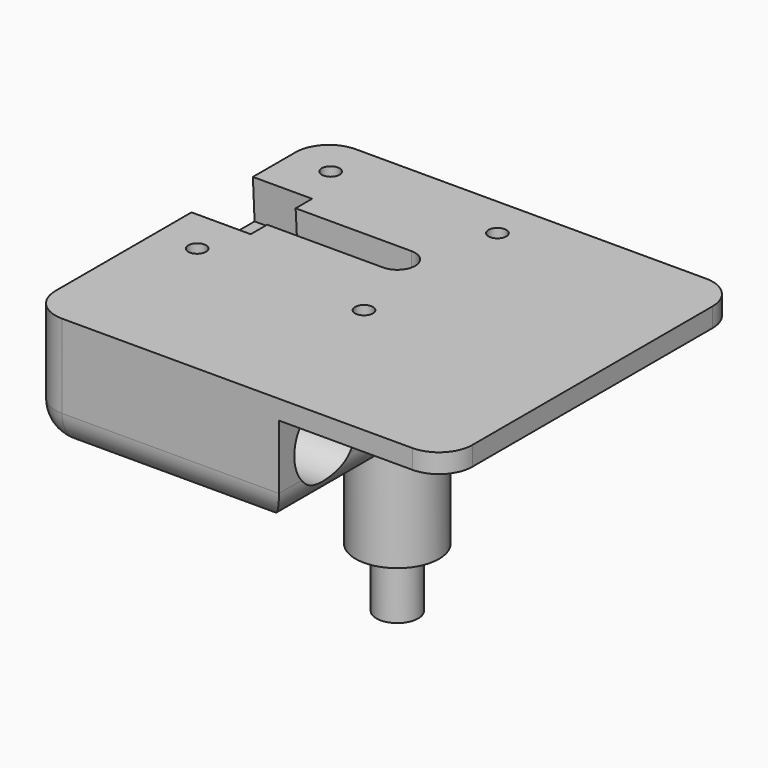
from build123d import *
from build123d import SkipClean  # not in build123d's __all__

# Parameters (mm, degrees)
F0_W          = 38.1
F0_H          = 12.7
F1_DEPTH      = 19.05
F2_W          = 9.017
F2_H          = 3.1369
F2_H_2        = 5.4102
F3_DEPTH      = 6.096
F3_TAPER      = -3
F4_DEPTH      = 4.318
F5_DEPTH      = 12.7010001
F7_R          = 6.35
F7_R_2        = 2.7051
F8_DEPTH      = 25.4
F9_R          = 3.175
F9_R_2        = 2.7051
F10_DEPTH     = 9.017
F11_DEPTH     = 17.78
F12_DEPTH     = 5.08
F14_D         = 11.938
F14_DEPTH     = 25.4
F14_TIP       = 3.586537035
F15_W         = 55.88
F15_H         = 2.921
F16_DEPTH     = 25.4
F17_T1_DEPTH  = 25.4
F17_T3_DEPTH  = 28.321
F17_T5_DEPTH  = 45.72
F17_T7_DEPTH  = 45.72
F17_T9_DEPTH  = 81.28
F17_S13_W     = 5.08
F17_S13_H     = 5.08
F17_T14_DEPTH = 5.08
F17_S19_W     = 5.08
F17_S19_H     = 5.08
F17_T20_DEPTH = 5.08
F18_D         = 2.7051
F18_DEPTH     = 10.16
F18_TIP       = 0.8126940303


# Not quite as in the source:
# - a fillet or chamfer that OpenCascade refuses, or shapes differently, is made with other operations: its cross-section is extruded or revolved along the edge and cut away or added
# - after a boolean that leaves OpenCascade's solid faulty, fix() repairs it


with BuildPart() as f1:
    # F0 (on Front) → F1 (new body, symmetric)
    with BuildSketch(Plane.XZ):
        Rectangle(F0_W, F0_H)
    extrude(amount=F1_DEPTH, both=True)

    # F2 (on face) → F3 (cut)
    with BuildSketch(Plane.XY.offset(6.35)):
        with Locations((-14.5415, 4.27355)):
            Rectangle(F2_W, F2_H)
        with Locations((-14.5415, 0)):
            Rectangle(F2_W, F2_H_2)
        with Locations((-14.5415, -4.27355)):
            Rectangle(F2_W, F2_H)
    extrude(amount=-F3_DEPTH, taper=F3_TAPER, mode=Mode.SUBTRACT)

    # F2 (on face) → F4 (cut)
    with BuildSketch(Plane.XY.offset(6.35)):
        with Locations((-14.5415, 4.27355)):
            Rectangle(F2_W, F2_H)
        with Locations((-14.5415, -4.27355)):
            Rectangle(F2_W, F2_H)
        with BuildLine():
            Line((7.62, 2.7051), (1.8750079208, 2.7051))
            ThreePointArc((1.8750079208, 2.7051), (1.27, 0), (1.8750079208, -2.7051))
            Line((1.8750079208, -2.7051), (7.62, -2.7051))
            ThreePointArc((7.62, -2.7051), (4.9149, 0), (7.62, 2.7051))
        make_face()
        with BuildLine():
            ThreePointArc((1.8750079208, -2.7051), (1.27, 0), (1.8750079208, 2.7051))
            Line((1.8750079208, 2.7051), (-10.033, 2.7051))
            Line((-10.033, 2.7051), (-10.033, -2.7051))
            Line((-10.033, -2.7051), (1.8750079208, -2.7051))
        make_face()
        with Locations((-14.5415, 0)):
            Rectangle(F2_W, F2_H_2)
    extrude(amount=-F4_DEPTH, mode=Mode.SUBTRACT)

    # F2 (on face) → F5 (cut, through all)
    with BuildSketch(Plane.XY.offset(6.35)):
        with BuildLine():
            ThreePointArc((10.3251, 0), (9.5327945538, 1.9127945538), (7.62, 2.7051))
            ThreePointArc((7.62, 2.7051), (4.9149, 0), (7.62, -2.7051))
            ThreePointArc((7.62, -2.7051), (9.5327945538, -1.9127945538), (10.3251, 0))
        make_face()
    extrude(amount=-F5_DEPTH, mode=Mode.SUBTRACT)

    # F7 (on face) → F8 (join)
    with BuildSketch(Plane(origin=(0, 0, -6.35), x_dir=(1, 0, 0), z_dir=(0, 0, -1))):
        with Locations((7.62, 0)):
            Circle(F7_R)
        with Locations((7.62, 0)):
            Circle(F7_R_2, mode=Mode.SUBTRACT)
    with SkipClean():  # cleaning this boolean's faces spoils the solid; the shape is the same uncleaned
        extrude(amount=F8_DEPTH)

    # F9 (on face) → F10 (join)
    with BuildSketch(Plane(origin=(0, 0, -31.75), x_dir=(1, 0, 0), z_dir=(0, 0, -1))):
        with Locations((7.62, 0)):
            Circle(F9_R)
        with Locations((7.62, 0)):
            Circle(F9_R_2, mode=Mode.SUBTRACT)
    extrude(amount=F10_DEPTH)

    add(f1.part.fix(), mode=Mode.REPLACE)

    # F11 (add): a face of the model
    f11_faces = [f1.faces().sort_by_distance(p)[0] for p in [
        (0, -19.05, 0),
    ]]
    extrude(f11_faces, amount=F11_DEPTH)

    # F12 (add): faces of the model
    f12_faces = [f1.faces().sort_by_distance(p)[0] for p in [
        (-0.7285482759, 0, -6.35),
        (0, -27.94, -6.35),
    ]]
    extrude(f12_faces, amount=F12_DEPTH)

    # F14
    with Locations(Plane.YZ.offset(19.05)):
        with Locations((-27.94, -2.54)):
            Hole(F14_D / 2, depth=F14_DEPTH)
            with Locations((0, 0, -(F14_DEPTH + F14_TIP / 2))):  # 118° drill point
                Cone(0, F14_D / 2, F14_TIP, mode=Mode.SUBTRACT)

    # F15 (on face) → F16 (join)
    with BuildSketch(Plane.YZ.offset(19.05)):
        with Locations((-8.89, 4.8895)):
            Rectangle(F15_W, F15_H)
    extrude(amount=F16_DEPTH)

    # F17: fillet of radius 5.08 on 8 edges, made by hand

    # F17_s2 → F17_t1 (cut)
    with BuildSketch(Plane.XY.offset(-6.35)):
        with BuildLine():
            ThreePointArc((-13.97, -36.83), (-17.5621024484, -35.3421024484), (-19.05, -31.75))
            Line((-19.05, -31.75), (-19.05, -36.83))
            Line((-19.05, -36.83), (-13.97, -36.83))
        make_face()
        with BuildLine():
            ThreePointArc((-13.97, 19.05), (-17.5621024484, 17.5621024484), (-19.05, 13.97))
            Line((-19.05, 13.97), (-19.05, 19.05))
            Line((-19.05, 19.05), (-13.97, 19.05))
        make_face()
    extrude(amount=F17_T1_DEPTH, mode=Mode.SUBTRACT)

    # F17_s4 → F17_t3 (cut)
    with BuildSketch(Plane.XY.offset(-9.271)):
        with BuildLine():
            ThreePointArc((39.37, 19.05), (42.9621024484, 17.5621024484), (44.45, 13.97))
            Line((44.45, 13.97), (44.45, 19.05))
            Line((44.45, 19.05), (39.37, 19.05))
        make_face()
        with BuildLine():
            ThreePointArc((44.45, -31.75), (42.9621024484, -35.3421024484), (39.37, -36.83))
            Line((39.37, -36.83), (44.45, -36.83))
            Line((44.45, -36.83), (44.45, -31.75))
        make_face()
    extrude(amount=F17_T3_DEPTH, mode=Mode.SUBTRACT)

    # F17_s6 → F17_t5 (cut)
    with BuildSketch(Plane.XZ.offset(-13.97)):
        with BuildLine():
            ThreePointArc((-13.97, -11.43), (-17.5621024484, -9.9421024484), (-19.05, -6.35))
            Line((-19.05, -6.35), (-19.05, -11.43))
            Line((-19.05, -11.43), (-13.97, -11.43))
        make_face()
    extrude(amount=F17_T5_DEPTH, mode=Mode.SUBTRACT)

    # F17_s8 → F17_t7 (cut)
    with BuildSketch(Plane.YZ.offset(-13.97)):
        with BuildLine():
            ThreePointArc((-31.75, -11.43), (-35.3421024484, -9.9421024484), (-36.83, -6.35))
            Line((-36.83, -6.35), (-36.83, -11.43))
            Line((-36.83, -11.43), (-31.75, -11.43))
        make_face()
        with BuildLine():
            ThreePointArc((13.97, -11.43), (17.5621024484, -9.9421024484), (19.05, -6.35))
            Line((19.05, -6.35), (19.05, -11.43))
            Line((19.05, -11.43), (13.97, -11.43))
        make_face()
    extrude(amount=F17_T7_DEPTH, mode=Mode.SUBTRACT)

    # F17_s10 → F17_t9 (cut)
    with BuildSketch(Plane.XZ.offset(-31.75)):
        with BuildLine():
            ThreePointArc((13.97, -11.43), (17.5621024484, -9.9421024484), (19.05, -6.35))
            Line((19.05, -6.35), (19.05, -11.43))
            Line((19.05, -11.43), (13.97, -11.43))
        make_face()
    extrude(amount=F17_T9_DEPTH, mode=Mode.SUBTRACT)


with BuildPart() as f17_tool12:
    # F17_s13 → F17_t14 (new body)
    with BuildSketch(Plane.XY.offset(-6.35)):
        with Locations((-16.51, -34.29)):
            Rectangle(F17_S13_W, F17_S13_H)
    extrude(amount=-F17_T14_DEPTH)

    # F17_s15 → F17_t16 (revolve, cut)
    with BuildSketch(Plane(origin=(-13.97, -31.75, -6.35), x_dir=(0.7071067812, 0.7071067812, 0), z_dir=(-0.7071067812, 0.7071067812, 0))):
        with BuildLine():
            ThreePointArc((0, -5.08), (5.08, 0), (0, 5.08))
            Line((0, 5.08), (0, -5.08))
        make_face()
    revolve(axis=Axis((-13.97, -31.75, -6.35), (0, 0, -1)), mode=Mode.SUBTRACT)


with BuildPart() as f1_1:
    add(f1.part, clean=False)

    # F17_t11: cut F17_tool12
    add(f17_tool12.part, mode=Mode.SUBTRACT)


with BuildPart() as f17_tool18:
    # F17_s19 → F17_t20 (new body)
    with BuildSketch(Plane.XZ.offset(-13.97)):
        with Locations((-16.51, -8.89)):
            Rectangle(F17_S19_W, F17_S19_H)
    extrude(amount=-F17_T20_DEPTH)

    # F17_s21 → F17_t22 (revolve, cut)
    with BuildSketch(Plane(origin=(-13.97, 13.97, -6.35), x_dir=(0.7071067812, 0, 0.7071067812), z_dir=(-0.7071067812, 0, 0.7071067812))):
        with BuildLine():
            ThreePointArc((0, -5.08), (5.08, 0), (0, 5.08))
            Line((0, 5.08), (0, -5.08))
        make_face()
    revolve(axis=Axis((-13.97, 13.97, -6.35), (0, 1, 0)), mode=Mode.SUBTRACT)


with BuildPart() as f1_2:
    add(f1_1.part, clean=False)

    # F17_t17: cut F17_tool18
    add(f17_tool18.part, mode=Mode.SUBTRACT)

    # F18
    with Locations(Plane.XY.offset(6.35)):
        with Locations((-12.7, 12.7), (-12.7, -12.7), (12.7, -12.7), (12.7, 12.7)):
            Hole(F18_D / 2, depth=F18_DEPTH)
            with Locations((0, 0, -(F18_DEPTH + F18_TIP / 2))):  # 118° drill point
                Cone(0, F18_D / 2, F18_TIP, mode=Mode.SUBTRACT)


solid = f1_2.part
